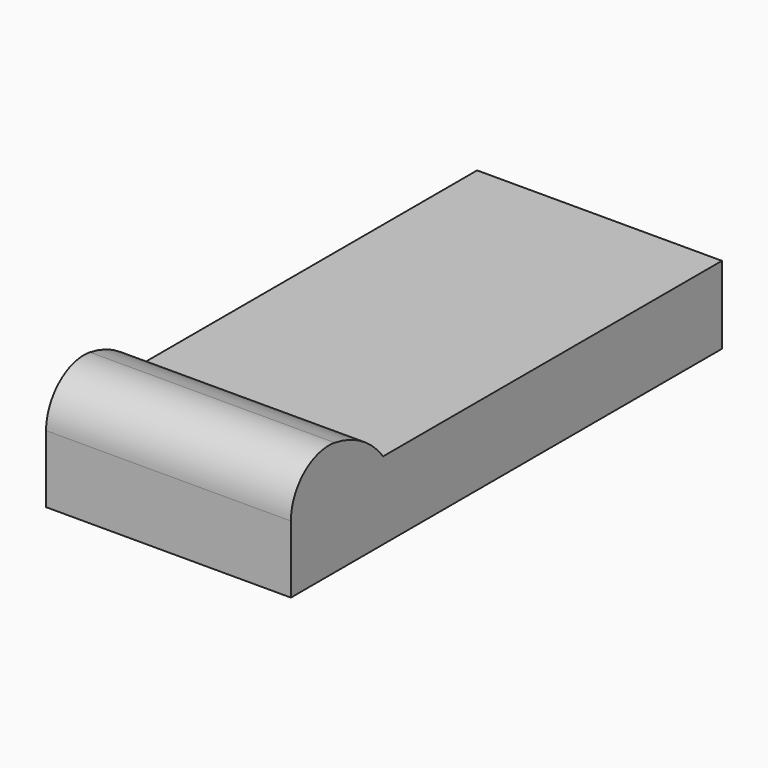
from build123d import *

# Parameters (mm, degrees)
F0_W        = 25.9
F0_H        = 57
F1_DEPTH    = 8.2
F2_W        = 25.9
F2_H        = 12.2
F3_DEPTH    = 4
F4_T1_DEPTH = 65.9
F5_R        = 5


# Not quite as in the source:
# - a fillet or chamfer that OpenCascade refuses, or shapes differently, is made with other operations: its cross-section is extruded or revolved along the edge and cut away or added


with BuildPart() as f1:
    # F0 (on Top) → F1 (new body)
    with BuildSketch(Plane.XY):
        with Locations((8.0425532069, 7.3918554072)):
            Rectangle(F0_W, F0_H)
    extrude(amount=F1_DEPTH)

    # F2 (on face) → F3 (join)
    with BuildSketch(Plane.XY.offset(8.2)):
        with Locations((8.0425532069, -15.0081445928)):
            Rectangle(F2_W, F2_H)
    extrude(amount=F3_DEPTH)

    # F4: fillet of radius 10 on 1 edges, made by hand

    # F4_s2 → F4_t1 (cut)
    with BuildSketch(Plane.YZ.offset(-24.9074467931)):
        with BuildLine():
            ThreePointArc((-8.9081445928, 8.2), (-12.4360086378, 11.14427191), (-16.9081445928, 12.2))
            Line((-16.9081445928, 12.2), (-8.9081445928, 12.2))
            Line((-8.9081445928, 12.2), (-8.9081445928, 8.2))
        make_face()
    extrude(amount=F4_T1_DEPTH, mode=Mode.SUBTRACT)

    # F5
    f5_edges = [f1.edges().sort_by_distance(p)[0] for p in [
        (8.042553, -21.108145, 12.2),
    ]]
    fillet(f5_edges, radius=F5_R)


solid = f1.part
